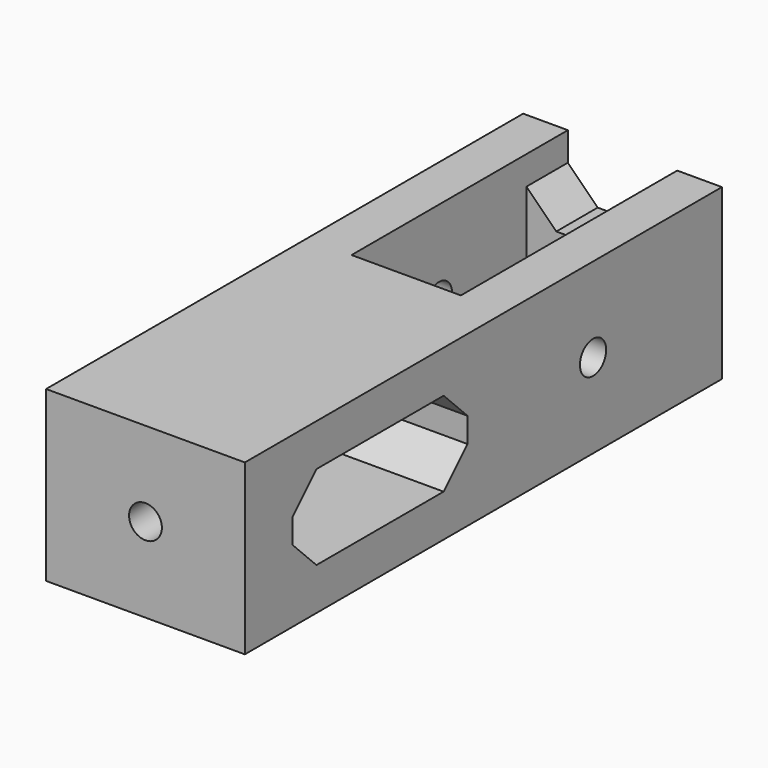
from build123d import *

# Parameters (mm, degrees)
F0_W          = 60
F0_H          = 17
F1_DEPTH      = 10
F2_W          = 22
F2_H          = 8.5
F3_DEPTH      = 25
F4_W          = 11
F4_H          = 22
F5_DEPTH      = 25
F6_R          = 1.65
F7_DEPTH      = 25
F8_W          = 11
F8_H          = 5.8824277986
F9_DEPTH      = 6
F10_SIZE      = 3
F12_DEPTH     = 1.5
F13_R         = 1.65
F14_DEPTH     = 10
F15_T1_DEPTH  = 20
F15_T6_DEPTH  = 20
F15_T12_DEPTH = 20
F15_T18_DEPTH = 20
F15_T25_DEPTH = 20
F15_T31_DEPTH = 20
F15_T37_DEPTH = 20
F15_T43_DEPTH = 20
F15_T49_DEPTH = 20
F15_T56_DEPTH = 20
F15_T62_DEPTH = 20


# Not quite as in the source:
# - a fillet or chamfer that OpenCascade refuses, or shapes differently, is made with other operations: its cross-section is extruded or revolved along the edge and cut away or added


with BuildPart() as f1:
    # F0 (on Right) → F1 (new body, symmetric)
    with BuildSketch(Plane.YZ):
        Rectangle(F0_W, F0_H)
    extrude(amount=F1_DEPTH, both=True)

    # F2 (on face) → F3 (cut)
    with BuildSketch(Plane.YZ.offset(10)):
        with Locations((-13, 0)):
            Rectangle(F2_W, F2_H)
    extrude(amount=-F3_DEPTH, mode=Mode.SUBTRACT)

    # F4 (on face) → F5 (cut)
    with BuildSketch(Plane.XY.offset(8.5)):
        with Locations((0, 13.7926964089)):
            Rectangle(F4_W, F4_H)
    extrude(amount=-F5_DEPTH, mode=Mode.SUBTRACT)

    # F6 (on face) → F7 (cut)
    with BuildSketch(Plane(origin=(-10, 0, 0), x_dir=(0, -1, 0), z_dir=(-1, 0, 0))):
        with Locations((-13.7926964089, 0)):
            Circle(F6_R)
    extrude(amount=-F7_DEPTH, mode=Mode.SUBTRACT)

    # F8 (on face) → F9 (cut)
    with BuildSketch(Plane(origin=(0, 30, 0), x_dir=(-1, 0, 0), z_dir=(0, 1, 0))):
        with Locations((0, 5.5587861007)):
            Rectangle(F8_W, F8_H)
        with Locations((0, -5.5587861007)):
            Rectangle(F8_W, F8_H)
    extrude(amount=-F9_DEPTH, mode=Mode.SUBTRACT)

    # F10
    f10_edges = [f1.edges().sort_by_distance(p)[0] for p in [
        (-5.5, 27.396348, 2.617572),
        (5.5, 27.396348, 2.617572),
        (5.5, 27.396348, -2.617572),
        (-5.5, 27.396348, -2.617572),
    ]]
    chamfer(f10_edges, length=F10_SIZE)

    # F11 (on face) → F12 (cut, symmetric)
    with BuildSketch(Plane(origin=(0, -24, 0), x_dir=(-1, 0, 0), z_dir=(0, 1, 0))):
        Polygon((-1.7320508076, 3), (-3.4641016151, 0), (-1.7320508076, -3), (1.7320508076, -3), (3.4641016151, 0), (1.7320508076, 3), align=None)
    extrude(amount=F12_DEPTH, both=True, mode=Mode.SUBTRACT)

    # F13 (on face) → F14 (cut)
    with BuildSketch(Plane.XZ.offset(30)):
        Circle(F13_R)
    extrude(amount=-F14_DEPTH, mode=Mode.SUBTRACT)

    # F15: chamfer of 3 on 4 edges, made by hand

    # F15_s2 → F15_t1 (join)
    with BuildSketch(Plane.YZ.offset(-10)):
        Polygon((-2, 1.25), (-5, 4.25), (-2, 4.25), align=None)
        Polygon((-5, -4.25), (-2, -1.25), (-2, -4.25), align=None)
    extrude(amount=F15_T1_DEPTH)


with BuildPart() as f15_tool4:
    # F15_s5 → F15_t6 (new body)
    with BuildSketch(Plane.YZ.offset(10)):
        Polygon((-21, -4.25), (-24, -1.25), (-24, -4.25), align=None)
    extrude(amount=-F15_T6_DEPTH)

    split(bisect_by=Plane.XY.offset(-3), keep=Keep.BOTTOM)

    split(bisect_by=Plane(origin=(2.5980762114, 0, -1.5), x_dir=(0, 1, 0), z_dir=(0.8660254038, 0, -0.5)), keep=Keep.TOP)


with BuildPart() as f1_1:
    add(f1.part)

    # F15_t3: union F15_tool4
    add(f15_tool4.part)


with BuildPart() as f15_tool10:
    # F15_s11 → F15_t12 (new body)
    with BuildSketch(Plane.YZ.offset(10)):
        Polygon((-21, -4.25), (-24, -1.25), (-24, -4.25), align=None)
    extrude(amount=-F15_T12_DEPTH)

    split(bisect_by=Plane.XY.offset(-3), keep=Keep.TOP)

    split(bisect_by=Plane(origin=(2.5980762114, 0, -1.5), x_dir=(0, 1, 0), z_dir=(0.8660254038, 0, -0.5)), keep=Keep.TOP)


with BuildPart() as f1_2:
    add(f1_1.part)

    # F15_t9: union F15_tool10
    add(f15_tool10.part)


with BuildPart() as f15_tool16:
    # F15_s17 → F15_t18 (new body)
    with BuildSketch(Plane.YZ.offset(10)):
        Polygon((-21, -4.25), (-24, -1.25), (-24, -4.25), align=None)
    extrude(amount=-F15_T18_DEPTH)

    split(bisect_by=Plane(origin=(-2.5980762114, 0, -1.5), x_dir=(0, 1, 0), z_dir=(0.8660254038, 0, 0.5)), keep=Keep.TOP)

    split(bisect_by=Plane.XY.offset(-3), keep=Keep.BOTTOM)

    split(bisect_by=Plane(origin=(2.5980762114, 0, -1.5), x_dir=(0, 1, 0), z_dir=(-0.8660254038, 0, 0.5)), keep=Keep.TOP)


with BuildPart() as f1_3:
    add(f1_2.part)

    # F15_t15: union F15_tool16
    add(f15_tool16.part)


with BuildPart() as f15_tool23:
    # F15_s24 → F15_t25 (new body)
    with BuildSketch(Plane.YZ.offset(10)):
        Polygon((-21, -4.25), (-24, -1.25), (-24, -4.25), align=None)
    extrude(amount=-F15_T25_DEPTH)

    split(bisect_by=Plane(origin=(-2.5980762114, 0, -1.5), x_dir=(0, 1, 0), z_dir=(-0.8660254038, 0, -0.5)), keep=Keep.TOP)

    split(bisect_by=Plane.XY.offset(-3), keep=Keep.BOTTOM)


with BuildPart() as f1_4:
    add(f1_3.part)

    # F15_t22: union F15_tool23
    add(f15_tool23.part)


with BuildPart() as f15_tool29:
    # F15_s30 → F15_t31 (new body)
    with BuildSketch(Plane.YZ.offset(10)):
        Polygon((-21, -4.25), (-24, -1.25), (-24, -4.25), align=None)
    extrude(amount=-F15_T31_DEPTH)

    split(bisect_by=Plane(origin=(-2.5980762114, 0, -1.5), x_dir=(0, 1, 0), z_dir=(-0.8660254038, 0, -0.5)), keep=Keep.TOP)

    split(bisect_by=Plane.XY.offset(-3), keep=Keep.TOP)


with BuildPart() as f1_5:
    add(f1_4.part)

    # F15_t28: union F15_tool29
    add(f15_tool29.part)


with BuildPart() as f15_tool35:
    # F15_s36 → F15_t37 (new body)
    with BuildSketch(Plane.YZ.offset(10)):
        Polygon((-24, 1.25), (-21, 4.25), (-24, 4.25), align=None)
    extrude(amount=-F15_T37_DEPTH)

    split(bisect_by=Plane(origin=(2.5980762114, 0, 1.5), x_dir=(0, 1, 0), z_dir=(0.8660254038, 0, 0.5)), keep=Keep.TOP)

    split(bisect_by=Plane.XY.offset(3), keep=Keep.BOTTOM)


with BuildPart() as f1_6:
    add(f1_5.part)

    # F15_t34: union F15_tool35
    add(f15_tool35.part)


with BuildPart() as f15_tool41:
    # F15_s42 → F15_t43 (new body)
    with BuildSketch(Plane.YZ.offset(10)):
        Polygon((-24, 1.25), (-21, 4.25), (-24, 4.25), align=None)
    extrude(amount=-F15_T43_DEPTH)

    split(bisect_by=Plane(origin=(2.5980762114, 0, 1.5), x_dir=(0, 1, 0), z_dir=(0.8660254038, 0, 0.5)), keep=Keep.TOP)

    split(bisect_by=Plane.XY.offset(3), keep=Keep.TOP)


with BuildPart() as f1_7:
    add(f1_6.part)

    # F15_t40: union F15_tool41
    add(f15_tool41.part)


with BuildPart() as f15_tool47:
    # F15_s48 → F15_t49 (new body)
    with BuildSketch(Plane.YZ.offset(10)):
        Polygon((-24, 1.25), (-21, 4.25), (-24, 4.25), align=None)
    extrude(amount=-F15_T49_DEPTH)

    split(bisect_by=Plane(origin=(-2.5980762114, 0, 1.5), x_dir=(0, 1, 0), z_dir=(0.8660254038, 0, -0.5)), keep=Keep.TOP)

    split(bisect_by=Plane(origin=(2.5980762114, 0, 1.5), x_dir=(0, 1, 0), z_dir=(-0.8660254038, 0, -0.5)), keep=Keep.TOP)

    split(bisect_by=Plane.XY.offset(3), keep=Keep.TOP)


with BuildPart() as f1_8:
    add(f1_7.part)

    # F15_t46: union F15_tool47
    add(f15_tool47.part)


with BuildPart() as f15_tool54:
    # F15_s55 → F15_t56 (new body)
    with BuildSketch(Plane.YZ.offset(10)):
        Polygon((-24, 1.25), (-21, 4.25), (-24, 4.25), align=None)
    extrude(amount=-F15_T56_DEPTH)

    split(bisect_by=Plane(origin=(-2.5980762114, 0, 1.5), x_dir=(0, 1, 0), z_dir=(-0.8660254038, 0, 0.5)), keep=Keep.TOP)

    split(bisect_by=Plane.XY.offset(3), keep=Keep.BOTTOM)


with BuildPart() as f1_9:
    add(f1_8.part)

    # F15_t53: union F15_tool54
    add(f15_tool54.part)


with BuildPart() as f15_tool60:
    # F15_s61 → F15_t62 (new body)
    with BuildSketch(Plane.YZ.offset(10)):
        Polygon((-24, 1.25), (-21, 4.25), (-24, 4.25), align=None)
    extrude(amount=-F15_T62_DEPTH)

    split(bisect_by=Plane(origin=(-2.5980762114, 0, 1.5), x_dir=(0, 1, 0), z_dir=(-0.8660254038, 0, 0.5)), keep=Keep.TOP)

    split(bisect_by=Plane.XY.offset(3), keep=Keep.TOP)


with BuildPart() as f1_10:
    add(f1_9.part)

    # F15_t59: union F15_tool60
    add(f15_tool60.part)


solid = f1_10.part
